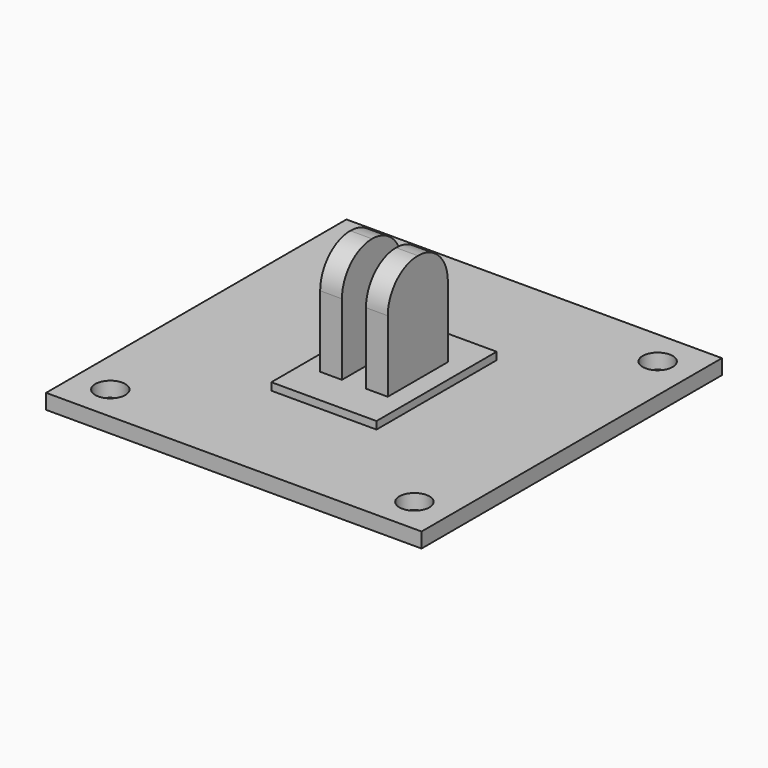
from build123d import *

# Parameters (mm, degrees)
F0_W     = 50
F0_H     = 50
F1_DEPTH = 2
F2_R     = 2
F3_DEPTH = 2
F4_W     = 14
F4_H     = 20
F5_DEPTH = 1
F6_W     = 2.9
F6_H     = 10
F7_DEPTH = 14.5
F8_R     = 4.99999


# Not quite as in the source:
# - a fillet or chamfer is up to 0.001 mm smaller than in the source, because OpenCascade refuses the exact size


with BuildPart() as f1:
    # F0 (on Top) → F1 (new body)
    with BuildSketch(Plane.XY):
        Rectangle(F0_W, F0_H)
    extrude(amount=F1_DEPTH)

    # F2 (on face) → F3 (cut)
    with BuildSketch(Plane.XY.offset(2)):
        with Locations((-20.25, 20.25)):
            Circle(F2_R)
        with Locations((20.25, 20.25)):
            Circle(F2_R)
        with Locations((20.25, -20.25)):
            Circle(F2_R)
        with Locations((-20.25, -20.25)):
            Circle(F2_R)
    extrude(amount=-F3_DEPTH, mode=Mode.SUBTRACT)

    # F4 (on face) → F5 (join)
    with BuildSketch(Plane.XY.offset(2)):
        Rectangle(F4_W, F4_H)
    extrude(amount=F5_DEPTH)

    # F6 (on face) → F7 (join)
    with BuildSketch(Plane.XY.offset(3)):
        with Locations((3.05, 0)):
            Rectangle(F6_W, F6_H)
        with Locations((-3.05, 0)):
            Rectangle(F6_W, F6_H)
    extrude(amount=F7_DEPTH)

    # F8 (radius 5 in the source; OpenCascade refuses exactly that, so slightly less here)
    f8_edges = [f1.edges().sort_by_distance(p)[0] for p in [
        (-3.05, 5, 17.5),
        (3.05, 5, 17.5),
        (3.05, -5, 17.5),
        (-3.05, -5, 17.5),
    ]]
    fillet(f8_edges, radius=F8_R)


solid = f1.part
